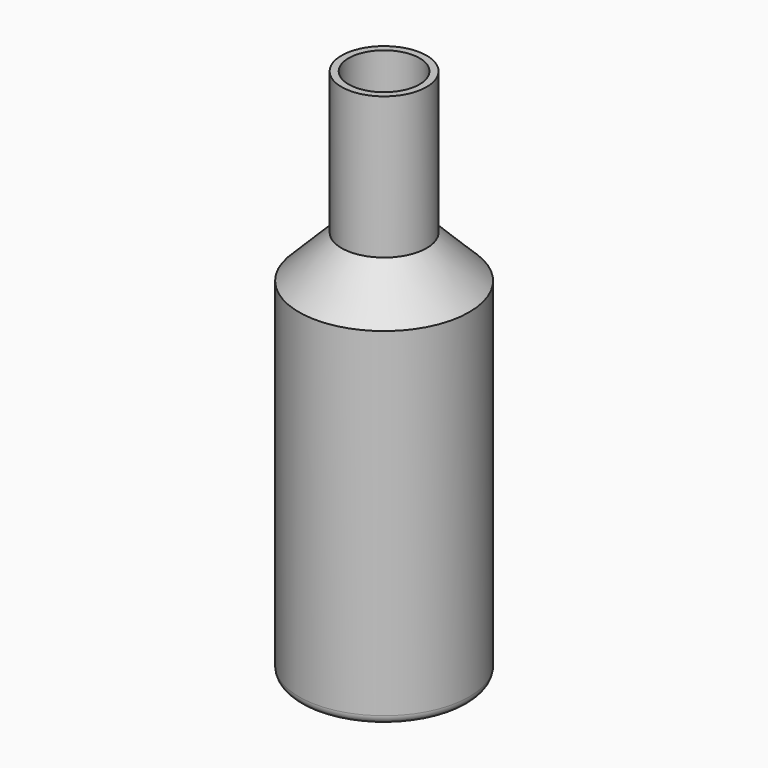
from build123d import *

# Parameters (mm, degrees)
F2_R = 2.54
F3_T = -2


with BuildPart() as f1:
    # F0 (on Front) → F1 (revolve)
    with BuildSketch(Plane.XZ):
        Polygon((0, 150.7095229592), (0, 0.7095229592), (24, 0.7095229592), (24, 98.7095229592), (12, 110.7095229592), (12, 150.7095229592), align=None)
    revolve(axis=Axis((0, 0, 75.7095229592), (0, 0, -1)))

    # F2
    f2_edges = [f1.edges().sort_by_distance(p)[0] for p in [
        (-24, 0, 0.709523),
    ]]
    fillet(f2_edges, radius=F2_R)

    # F3
    f3_openings = [f1.faces().sort_by_distance(p)[0] for p in [
        (0, 0, 150.709523),
    ]]
    offset(amount=F3_T, openings=f3_openings, kind=Kind.INTERSECTION)


solid = f1.part
